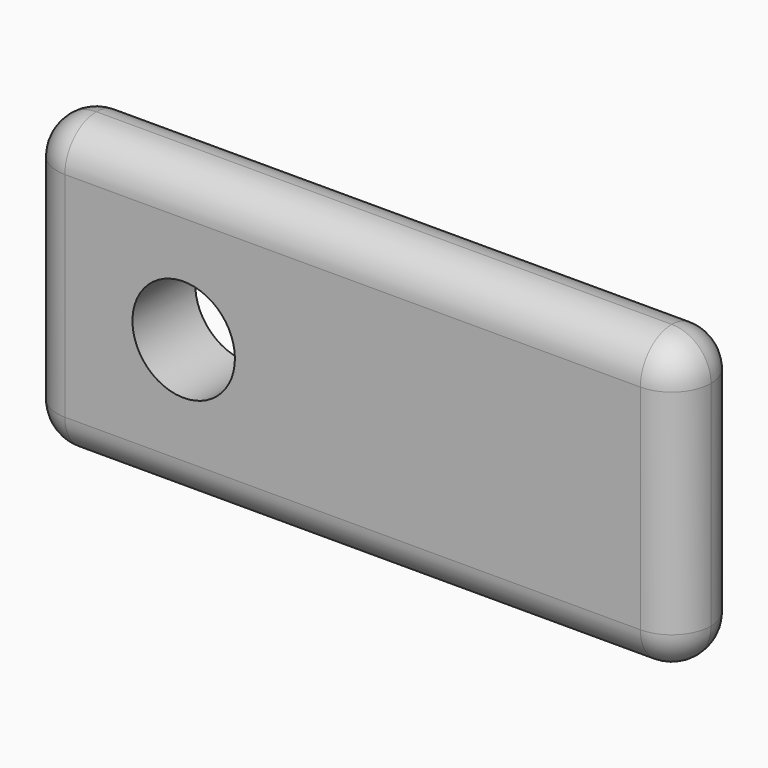
from build123d import *

# Parameters (mm, degrees)
F1_DEPTH = 4.572
F2_R     = 2.28599


# Not quite as in the source:
# - a fillet or chamfer is up to 0.001 mm smaller than in the source, because OpenCascade refuses the exact size


with BuildPart() as f1:
    # F0 (on Front) → F1 (new body)
    with BuildSketch(Plane.XZ):
        with BuildLine():
            Line((-29.10264256, -17.6625937588), (-67.20264256, -17.6625937588))
            Line((-67.20264256, -17.6625937588), (-67.20264256, -26.1715937588))
            Line((-67.20264256, -26.1715937588), (-60.9790929348, -26.1715937588))
            ThreePointArc((-60.9790929348, -26.1715937588), (-57.9945929348, -23.1870937588), (-55.0100929348, -26.1715937588))
            Line((-55.0100929348, -26.1715937588), (-29.10264256, -26.1715937588))
            Line((-29.10264256, -26.1715937588), (-29.10264256, -17.6625937588))
        make_face()
        with BuildLine():
            Line((-60.9790929348, -26.1715937588), (-67.20264256, -26.1715937588))
            Line((-67.20264256, -26.1715937588), (-67.20264256, -34.6805937588))
            Line((-67.20264256, -34.6805937588), (-29.10264256, -34.6805937588))
            Line((-29.10264256, -34.6805937588), (-29.10264256, -26.1715937588))
            Line((-29.10264256, -26.1715937588), (-55.0100929348, -26.1715937588))
            ThreePointArc((-55.0100929348, -26.1715937588), (-57.9945929348, -29.1560937588), (-60.9790929348, -26.1715937588))
        make_face()
    extrude(amount=F1_DEPTH)

    # F2 (radius 2.286 in the source; OpenCascade refuses exactly that, so slightly less here)
    f2_edges = [f1.edges().sort_by_distance(p)[0] for p in [
        (-67.202643, -2.286, -17.662594),
        (-29.102643, -2.286, -17.662594),
        (-29.102643, -2.286, -34.680594),
        (-67.202643, -2.286, -34.680594),
        (-48.152643, -4.572, -34.680594),
        (-48.152643, 0, -34.680594),
        (-29.102643, 0, -26.171594),
        (-29.102643, -4.572, -26.171594),
        (-48.152643, -4.572, -17.662594),
        (-48.152643, 0, -17.662594),
        (-67.202643, 0, -26.171594),
        (-67.202643, -4.572, -26.171594),
    ]]
    fillet(f2_edges, radius=F2_R)


solid = f1.part
